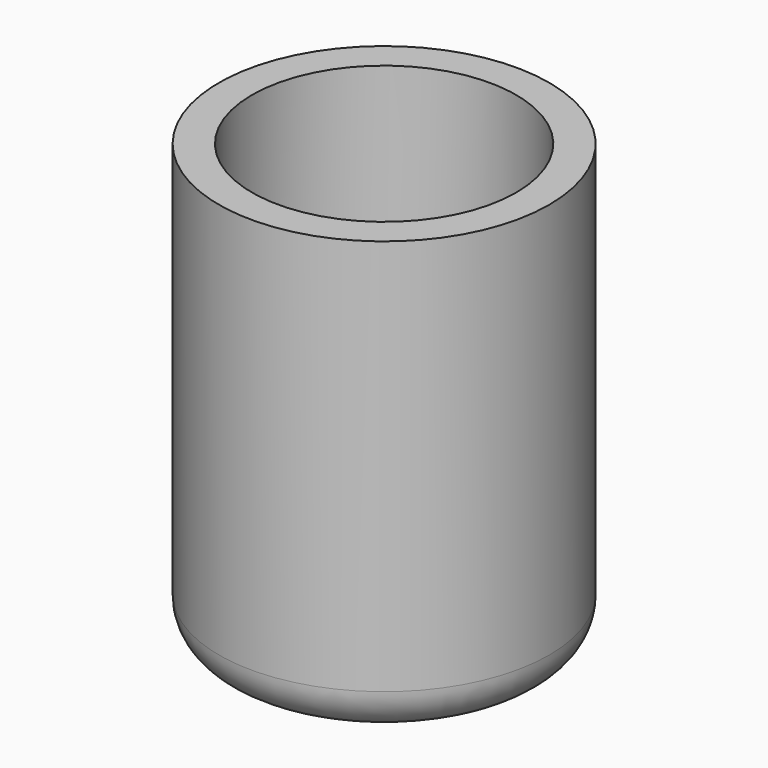
from build123d import *

# Parameters (mm, degrees)
F0_R        = 7.5
F1_DEPTH    = 10
F3_DEPTH    = 7
F5_DEPTH    = 1
F6_T2_ANGLE = 299.893258673
F6_T4_ANGLE = 119.7759847122
F2_R        = 7.5
F2_R_2      = 6
F7_DEPTH    = 5
F8_DEPTH    = 5


# Not quite as in the source:
# - a fillet or chamfer that OpenCascade refuses, or shapes differently, is made with other operations: its cross-section is extruded or revolved along the edge and cut away or added


with BuildPart() as f1:
    # F0 (on Top) → F1 (new body)
    with BuildSketch(Plane.XY):
        Circle(F0_R)
    extrude(amount=F1_DEPTH)

    # F2 (on face) → F3 (cut)
    with BuildSketch(Plane.XY.offset(10)):
        with BuildLine():
            Line((-4.4899339722, 0.3008204206), (4.4899339722, 0.3008204206))
            ThreePointArc((4.4899339722, 0.3008204206), (0, 4.5), (-4.4899339722, 0.3008204206))
        make_face()
        with BuildLine():
            ThreePointArc((-4.4955897828, -0.1991795794), (0, -4.5), (4.4955897828, -0.1991795794))
            Line((4.4955897828, -0.1991795794), (-4.4955897828, -0.1991795794))
        make_face()
    extrude(amount=-F3_DEPTH, mode=Mode.SUBTRACT)

    # F4 (on face) → F5 (cut)
    with BuildSketch(Plane(origin=(0, 0, 0), x_dir=(1, 0, 0), z_dir=(0, 0, -1))):
        with BuildLine():
            Line((-1.1, -1), (-1.1, -7.4188947964))
            ThreePointArc((-1.1, -7.4188947964), (0, -7.5), (1.1, -7.4188947964))
            Line((1.1, -7.4188947964), (1.1, -1))
            Line((1.1, -1), (0, -1))
            Line((0, -1), (-1.1, -1))
        make_face()
    extrude(amount=-F5_DEPTH, mode=Mode.SUBTRACT)

    # F6: fillet of radius 2 on 1 edges, made by hand

    # F6_s1 → F6_t2 (revolve, cut)
    with BuildSketch(Plane(origin=(0, 0, 0), x_dir=(0, 0, 1), z_dir=(0.8669553942, -0.4983857387, 0))):
        with BuildLine():
            ThreePointArc((2, -7.5), (0.5857864376, -6.9142135624), (0, -5.5))
            Line((0, -5.5), (0, -7.5))
            Line((0, -7.5), (2, -7.5))
        make_face()
    revolve(axis=Axis((0, 0, 0), (0, 0, 1)), revolution_arc=F6_T2_ANGLE, mode=Mode.SUBTRACT)

    # F6_s3 → F6_t4 (revolve, cut)
    with BuildSketch(Plane.XZ):
        with BuildLine():
            ThreePointArc((7.5, 2), (6.9142135624, 0.5857864376), (5.5, 0))
            Line((5.5, 0), (7.5, 0))
            Line((7.5, 0), (7.5, 2))
        make_face()
    revolve(axis=Axis((0, 0, 0), (0, 0, 1)), revolution_arc=F6_T4_ANGLE, mode=Mode.SUBTRACT)

    # F2 (on face) → F7 (join)
    with BuildSketch(Plane.XY.offset(10)):
        Circle(F2_R)
        Circle(F2_R_2, mode=Mode.SUBTRACT)
    extrude(amount=F7_DEPTH)

    # F8 (add): a face of the model
    f8_faces = [f1.faces().sort_by_distance(p)[0] for p in [
        (-7.2878679656, 0, 15),
    ]]
    extrude(f8_faces, amount=F8_DEPTH)


solid = f1.part
